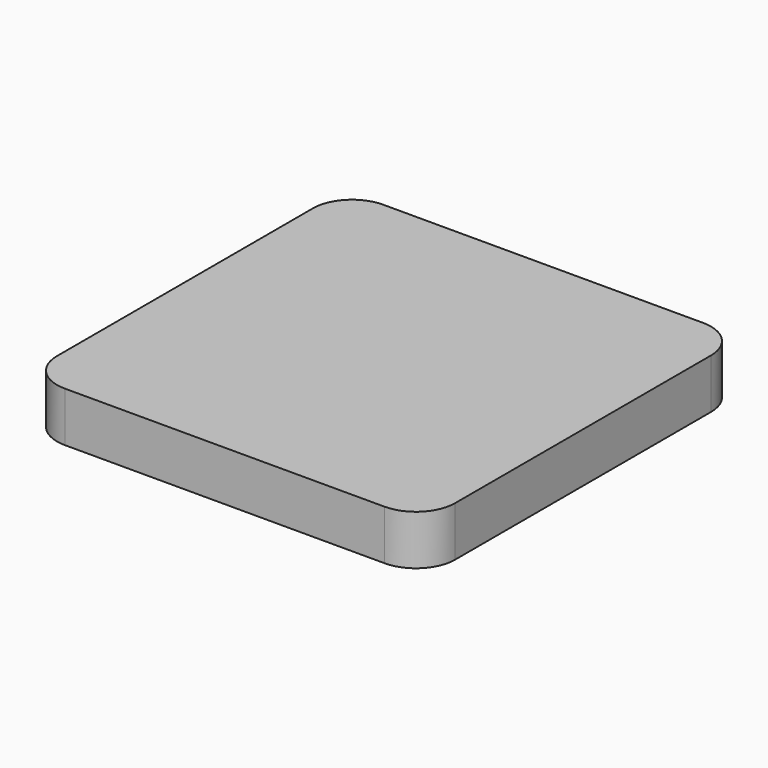
from build123d import *

# Parameters (mm, degrees)
F0_W     = 25.4
F0_H     = 25.4
F1_DEPTH = 3.175
F2_R     = 2.5


# Not quite as in the source:
# - a length typed as a fraction of an inch, garbled in the dataset ("3 / 203.2 mm" for 3/8 in), is restored


with BuildPart() as f1:
    # F0 (on Top) → F1 (new body)
    with BuildSketch(Plane.XY):
        Rectangle(F0_W, F0_H)
    extrude(amount=F1_DEPTH)

    # F2
    f2_edges = [f1.edges().sort_by_distance(p)[0] for p in [
        (12.7, -12.7, 1.5875),
        (-12.7, -12.7, 1.5875),
        (12.7, 12.7, 1.5875),
        (-12.7, 12.7, 1.5875),
    ]]
    fillet(f2_edges, radius=F2_R)


solid = f1.part
